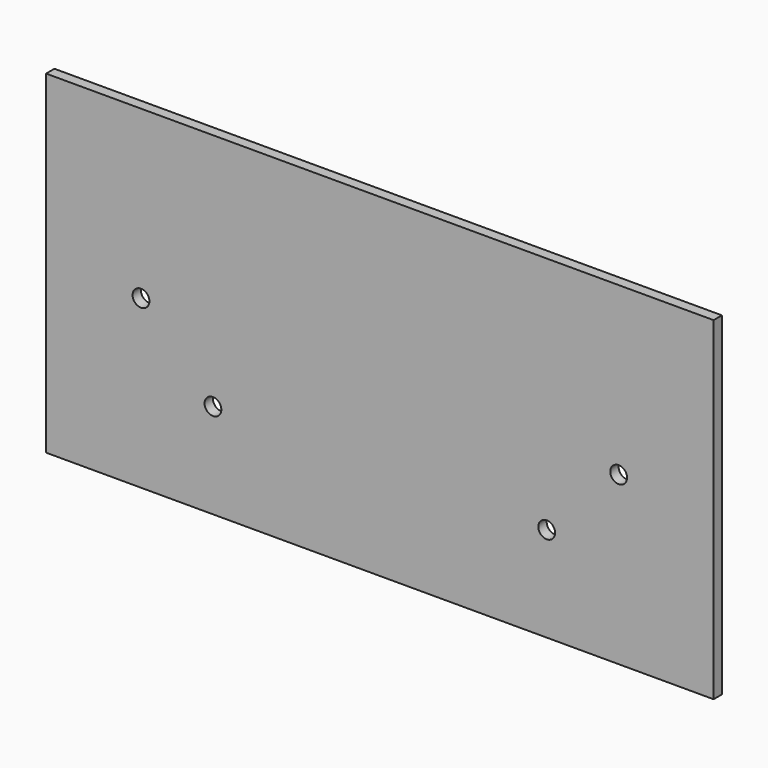
from build123d import *

# Parameters (mm, degrees)
F0_W     = 203.2
F0_H     = 101.6
F1_DEPTH = 3.175
F3_D     = 5.1054
F3_DEPTH = 25
F3_TIP   = 1.5338169022


# Not quite as in the source:
# - a length typed as a fraction of an inch, garbled in the dataset ("3 / 203.2 mm" for 3/8 in), is restored


with BuildPart() as f1:
    # F0 (on Front) → F1 (new body)
    with BuildSketch(Plane.XZ):
        Rectangle(F0_W, F0_H)
    extrude(amount=F1_DEPTH)

    # F3
    with Locations(Plane.XZ.offset(3.175)):
        with Locations((-50.8, -21.9075), (50.8, -21.9075), (-72.7075, 0), (72.7075, 0)):
            Hole(F3_D / 2, depth=F3_DEPTH)
            with Locations((0, 0, -(F3_DEPTH + F3_TIP / 2))):  # 118° drill point
                Cone(0, F3_D / 2, F3_TIP, mode=Mode.SUBTRACT)


solid = f1.part
